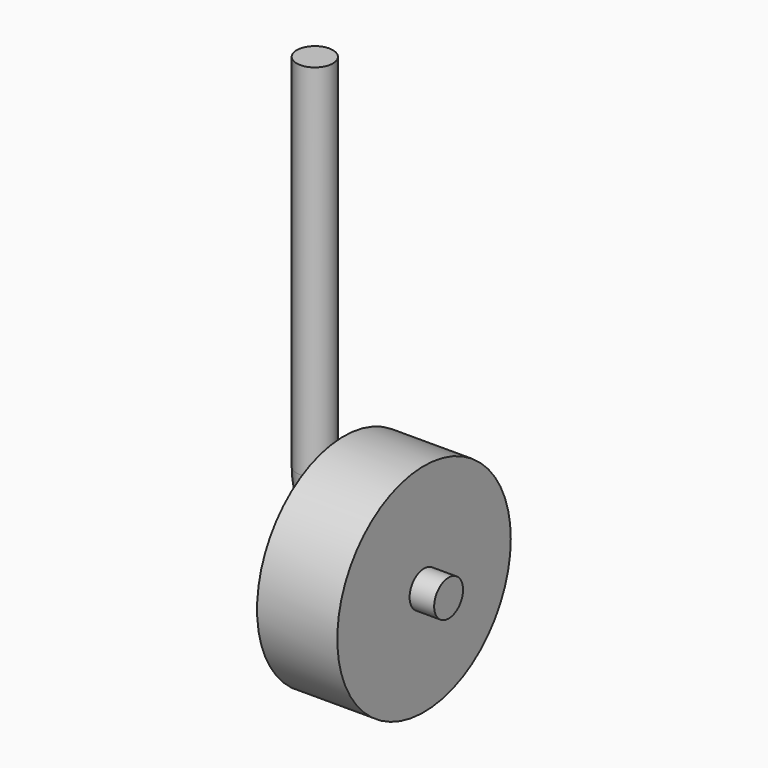
from build123d import *

# Parameters (mm, degrees)
F0_R      = 6.35
F1_DEPTH  = 101.6
F1_FACE_R = 6.35
F4_R      = 38.1
F4_R_2    = 6.35
F5_DEPTH  = 28.194
F6_R      = 6.35
F7_DEPTH  = 8.636


with BuildPart() as f1:
    # F0 (on Top) → F1 (new body)
    with BuildSketch(Plane.XY):
        Circle(F0_R)
    extrude(amount=-F1_DEPTH)

    # F3: sweep along a path in F2
    with BuildLine(Plane.XZ) as f3_path:
        Line((0, -100.055642426), (0, -126.7550863981))
        ThreePointArc((0, -126.7550863981), (7.4394877579, -144.7155986403), (25.4, -152.1550863981))
        Line((25.4, -152.1550863981), (38.380023092, -152.1550863981))
    # F1_face (on face) → F3 (sweep)
    with BuildSketch(Plane(origin=(0, 0, -101.6), x_dir=(1, 0, 0), z_dir=(0, 0, -1))):
        Circle(F1_FACE_R)
    sweep(path=f3_path.line)

    # F6 (on face) → F7 (join)
    with BuildSketch(Plane.YZ.offset(38.380023092)):
        with Locations((0, -152.1550863981)):
            Circle(F6_R)
    extrude(amount=F7_DEPTH)


with BuildPart() as f5:
    # F4 (on face) → F5 (new body)
    with BuildSketch(Plane.YZ.offset(38.380023092)):
        with Locations((0, -152.1550863981)):
            Circle(F4_R)
        with Locations((0, -152.1550863981)):
            Circle(F4_R_2, mode=Mode.SUBTRACT)
    extrude(amount=-F5_DEPTH)


solid = Compound([f1.part, f5.part])
